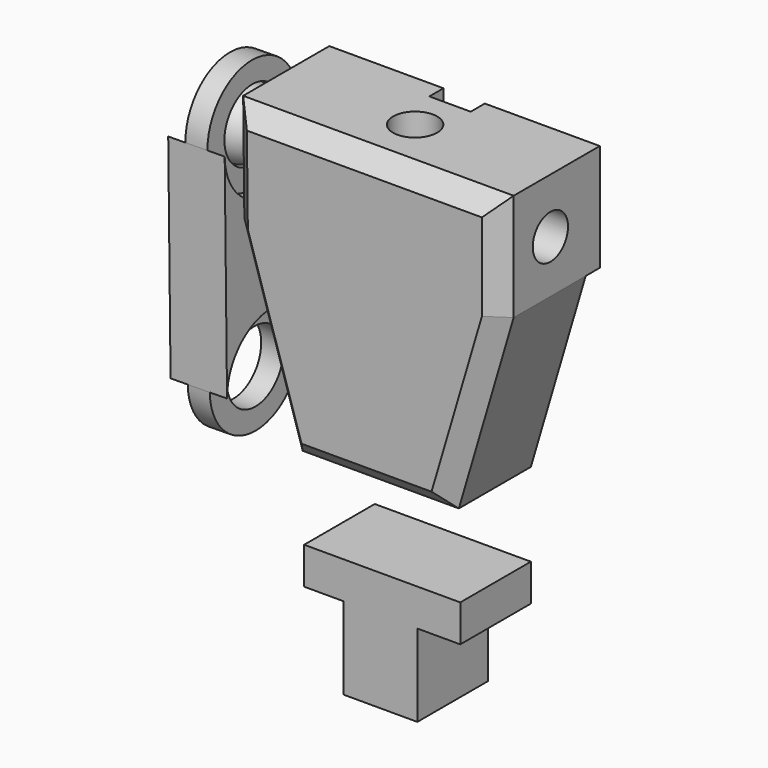
from build123d import *

# Parameters (mm, degrees)
F1_DEPTH  = 6.35
F2_R      = 3.175
F3_DEPTH  = 6.35
F4_R      = 3.175
F5_DEPTH  = 6.35
F6_R      = 3.175
F7_DEPTH  = 6.35
F8_R      = 3.175
F9_DEPTH  = 6.35
F11_DEPTH = 2.794
F12_SIZE  = 2.54
F14_DEPTH = 2.54
F17_DEPTH = 1.5875
F18_DEPTH = 4.064
F21_DEPTH = 9.144


with BuildPart() as f1:
    # F0 (on Front) → F1 (new body, symmetric)
    with BuildSketch(Plane.XZ):
        Polygon((19.4665305316, 46.8225739896), (-19.4665268064, 46.8225739896), (-19.2950163037, 31.3865616918), (-10.89096535, 4.6308040619), (11.5770100861, 4.6308040619), (19.4665305316, 31.3865616918), align=None)
    extrude(amount=F1_DEPTH, both=True)

    # F2 (on face) → F3 (cut)
    with BuildSketch(Plane(origin=(-18.9439395066, 0, -0.2104873024), x_dir=(0, -1, 0), z_dir=(-0.9999382779, 0, -0.011110377))):
        with Locations((0, 39.3174812198)):
            Circle(F2_R)
    extrude(amount=-F3_DEPTH, mode=Mode.SUBTRACT)

    # F4 (on face) → F5 (cut)
    with BuildSketch(Plane.YZ.offset(19.4665305316)):
        with Locations((0, 38.933057338)):
            Circle(F4_R)
    extrude(amount=-F5_DEPTH, mode=Mode.SUBTRACT)

    # F6 (on face) → F7 (cut)
    with BuildSketch(Plane.XY.offset(46.8225739896)):
        Circle(F6_R)
    extrude(amount=-F7_DEPTH, mode=Mode.SUBTRACT)

    # F8 (on face) → F9 (cut)
    with BuildSketch(Plane(origin=(0, 0, 4.6308040619), x_dir=(1, 0, 0), z_dir=(0, 0, -1))):
        Circle(F8_R)
    extrude(amount=-F9_DEPTH, mode=Mode.SUBTRACT)

    # F10 (on face) → F11 (join)
    with BuildSketch(Plane.XZ.offset(6.35)):
        Polygon((19.4665305316, 31.3865616918), (19.4665305316, 46.8225739896), (-19.4665268064, 46.8225739896), (-19.2950163037, 31.3865616918), (-10.89096535, 4.6308040619), (11.5770100861, 4.6308040619), align=None)
    extrude(amount=F11_DEPTH)

    # F12
    f12_edges = [f1.edges().sort_by_distance(p)[0] for p in [
        (-19.380772, -9.144, 39.104568),
        (19.466531, -9.144, 39.104568),
        (2e-06, -9.144, 46.822574),
        (0.343022, -9.144, 4.630804),
        (-15.092991, -9.144, 18.008683),
        (15.52177, -9.144, 18.008683),
    ]]
    chamfer(f12_edges, length=F12_SIZE)

    # F13 (on face) → F14 (join)
    with BuildSketch(Plane(origin=(0, 6.35, 0), x_dir=(-1, 0, 0), z_dir=(0, 1, 0))):
        Polygon((-19.4665305316, 46.8225739896), (-19.4665305316, 31.3865616918), (-5.9960167855, 31.3865616918), (-2.9173761141, 35.8410552144), (-2.9173761141, 46.8225739896), align=None)
        Polygon((19.4665268064, 46.8225739896), (3.034662921, 46.8225739896), (3.034662921, 35.8410552144), (6.523788441, 31.3865616918), (19.2950163037, 31.3865616918), align=None)
    extrude(amount=F14_DEPTH)


with BuildPart() as f1b:
    # F0 (on Front) → F1, piece 2 (new body, symmetric)
    with BuildSketch(Plane.XZ):
        Polygon((11.5770100861, -7.3749837466), (-10.89096535, -7.3749837466), (-10.89096535, -12.6918321475), (-5.2310945466, -12.6918321475), (-5.2310945466, -24.526109919), (5.402605515, -24.526109919), (5.402605515, -12.6918321475), (11.5770100861, -12.6918321475), align=None)
    extrude(amount=F1_DEPTH, both=True)


with BuildPart() as f17:
    # F16 (on offset) → F17 (new body, symmetric)
    with BuildSketch(Plane(origin=(-24.5315946033, 0, -0.2725720893), x_dir=(0, -1, 0), z_dir=(-0.9999382779, 0, -0.011110377))):
        with BuildLine():
            Line((5.08, 39.497371763), (8.128, 39.497371763))
            ThreePointArc((8.128, 39.497371763), (0, 47.625371763), (-8.128, 39.497371763))
            Line((-8.128, 39.497371763), (-5.08, 39.497371763))
            ThreePointArc((-5.08, 39.497371763), (0, 44.577371763), (5.08, 39.497371763))
        make_face()
        with BuildLine():
            ThreePointArc((-8.128, 39.497371763), (0, 31.369371763), (8.128, 39.497371763))
            Line((8.128, 39.497371763), (5.08, 39.497371763))
            ThreePointArc((5.08, 39.497371763), (0, 34.417371763), (-5.08, 39.497371763))
            Line((-5.08, 39.497371763), (-8.128, 39.497371763))
        make_face()
    extrude(amount=F17_DEPTH, both=True)



with BuildPart() as f17b:
    # F16 (on offset) → F17, piece 2 (new body, symmetric)
    with BuildSketch(Plane(origin=(-24.5315946033, 0, -0.2725720893), x_dir=(0, -1, 0), z_dir=(-0.9999382779, 0, -0.011110377))):
        with BuildLine():
            ThreePointArc((-8.128, 8.9525301009), (0, 0.8245301009), (8.128, 8.9525301009))
            Line((8.128, 8.9525301009), (5.08, 8.9525301009))
            ThreePointArc((5.08, 8.9525301009), (0, 3.8725301009), (-5.08, 8.9525301009))
            Line((-5.08, 8.9525301009), (-8.128, 8.9525301009))
        make_face()
        with BuildLine():
            Line((5.08, 8.9525301009), (8.128, 8.9525301009))
            ThreePointArc((8.128, 8.9525301009), (0, 17.0805301009), (-8.128, 8.9525301009))
            Line((-8.128, 8.9525301009), (-5.08, 8.9525301009))
            ThreePointArc((-5.08, 8.9525301009), (0, 14.0325301009), (5.08, 8.9525301009))
        make_face()
    extrude(amount=F17_DEPTH, both=True)


with BuildPart() as f17_1:
    add(f17.part)

    add(f17b.part)  # F18 merges F17b
    # F16 (on offset) → F18 (join, symmetric)
    with BuildSketch(Plane(origin=(-24.5315946033, 0, -0.2725720893), x_dir=(0, -1, 0), z_dir=(-0.9999382779, 0, -0.011110377))):
        with BuildLine():
            Line((8.128, 8.9525301009), (8.128, 39.497371763))
            ThreePointArc((8.128, 39.497371763), (0, 31.369371763), (-8.128, 39.497371763))
            Line((-8.128, 39.497371763), (-8.128, 8.9525301009))
            ThreePointArc((-8.128, 8.9525301009), (0, 17.0805301009), (8.128, 8.9525301009))
        make_face()
    extrude(amount=F18_DEPTH, both=True)


with BuildPart() as f20:
    # F19 (on offset) → F20 (revolve)
    with BuildSketch(Plane(origin=(-24.5315946033, 0, -0.2725720893), x_dir=(0, -1, 0), z_dir=(-0.9999382779, 0, -0.011110377))):
        with BuildLine():
            Line((0, 42.5922383981), (0, 44.4364689796))
            ThreePointArc((0, 44.4364689796), (-4.953, 39.4834689796), (0, 34.5304689796))
            Line((0, 34.5304689796), (0, 36.3746995611))
            ThreePointArc((0, 36.3746995611), (-3.1087694185, 39.4834689796), (0, 42.5922383981))
        make_face()
    revolve(axis=Axis((-24.9702708307, 0, 39.208459886), (0.011110377, 0, -0.9999382779)))

    # F19 (on offset) → F21 (join)
    with BuildSketch(Plane(origin=(-24.5315946033, 0, -0.2725720893), x_dir=(0, -1, 0), z_dir=(-0.9999382779, 0, -0.011110377))):
        with BuildLine():
            ThreePointArc((3.1087694185, 39.4834689796), (2.1982319369, 41.6817009165), (0, 42.5922383981))
            Line((0, 42.5922383981), (0, 36.3746995611))
            ThreePointArc((0, 36.3746995611), (2.1982319369, 37.2852370427), (3.1087694185, 39.4834689796))
        make_face()
        with BuildLine():
            Line((0, 36.3746995611), (0, 42.5922383981))
            ThreePointArc((0, 42.5922383981), (-3.1087694185, 39.4834689796), (0, 36.3746995611))
        make_face()
    extrude(amount=-F21_DEPTH)


solid = Compound([f1.part, f1b.part, f17_1.part, f20.part])
